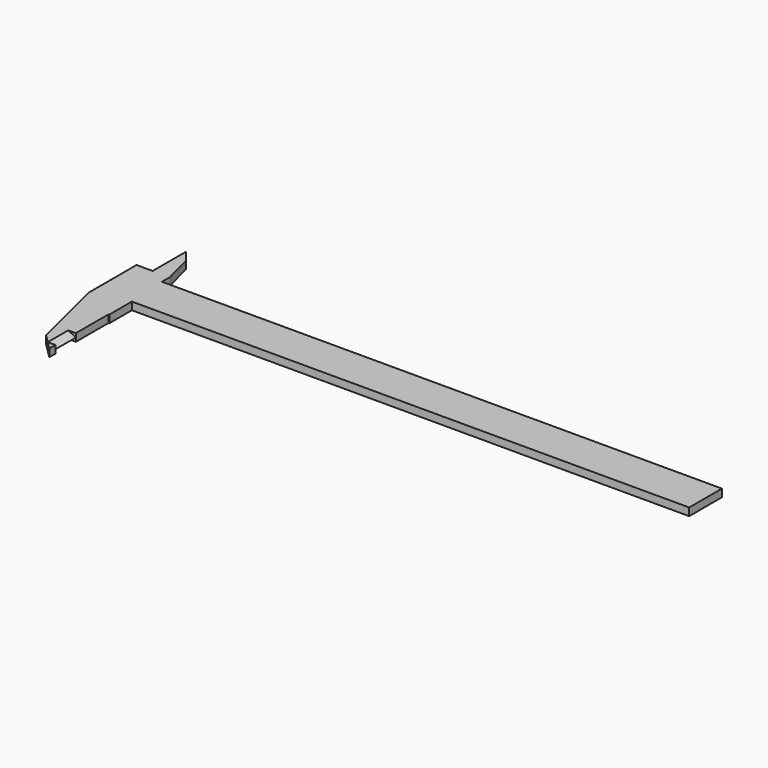
from build123d import *

# Parameters (mm, degrees)
F1_DEPTH = 3
F4_DEPTH = 10


# Not quite as in the source:
# - a feature names something its author has since deleted; it is built from what else it names


with BuildPart() as f1:
    # F0 (on Top) → F1 (new body)
    with BuildSketch(Plane.XY):
        Polygon((0, -16), (0, 0), (-219, 0), (-219, 3.8), (-222.0407651073, 15.5), (-225.7, 20), (-225.7, 3.8), (-232, 3.8), (-232, -19.5), (-224.5, -49.8), (-218.3, -56), (-218.3, -27), (-218, -27), (-218, -16), align=None)
    extrude(amount=F1_DEPTH)

    # F3 (on offset) → F4 (cut)
    with BuildSketch(Plane.XZ.offset(53)):
        Polygon((-221.3, 3), (-218.3, 1.5), (-221.3, 0), (-213.3, 0), (-213.3, 3), align=None)
    extrude(amount=-F4_DEPTH, mode=Mode.SUBTRACT)


solid = f1.part
